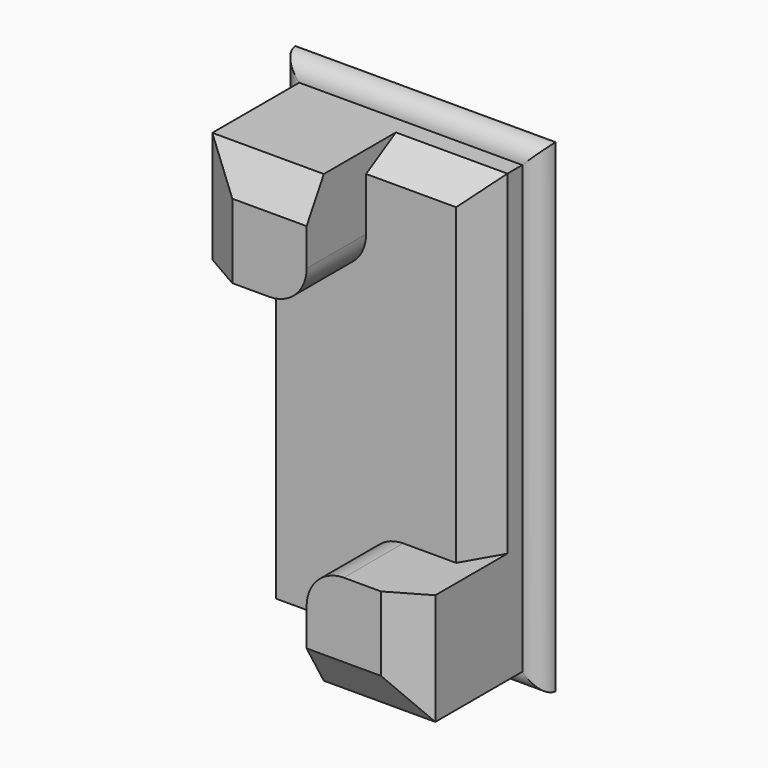
from build123d import *

# Parameters (mm, degrees)
F0_W       = 88.9
F0_H       = 165.1
F1_DEPTH   = 6.35
F2_DEPTH   = 25.4
F3_DEPTH   = 50.8
F4_SIZE2   = 7.3323484187
F4_SIZE    = 12.7
F4_2_SIZE2 = 7.3323484187
F4_2_SIZE  = 12.7
F5_R       = 6.34999
F6_SIZE2   = 7.3323484187
F6_SIZE    = 12.7
F7_SIZE2   = 7.3323484187
F7_SIZE    = 12.7


# Not quite as in the source:
# - a fillet or chamfer is up to 0.001 mm smaller than in the source, because OpenCascade refuses the exact size


with BuildPart() as f1:
    # F0 (on Front) → F1 (new body)
    with BuildSketch(Plane.XZ):
        Rectangle(F0_W, F0_H)
        Polygon((-38.1, 38.1), (-38.1, 76.2), (0, 76.2), (38.1, 76.2), (38.1, -38.1), (38.1, -76.2), (0, -76.2), (-38.1, -76.2), align=None, mode=Mode.SUBTRACT)
    extrude(amount=F1_DEPTH)

    # F0 (on Front) → F2 (join)
    with BuildSketch(Plane.XZ):
        with BuildLine():
            Line((38.1, 76.2), (0, 76.2))
            Line((0, 76.2), (0, 50.8))
            ThreePointArc((0, 50.8), (-3.7197438789, 41.8197438789), (-12.7, 38.1))
            Line((-12.7, 38.1), (-38.1, 38.1))
            Line((-38.1, 38.1), (-38.1, -76.2))
            Line((-38.1, -76.2), (0, -76.2))
            Line((0, -76.2), (0, -50.8))
            ThreePointArc((0, -50.8), (3.7197438789, -41.8197438789), (12.7, -38.1))
            Line((12.7, -38.1), (38.1, -38.1))
            Line((38.1, -38.1), (38.1, 76.2))
        make_face()
    extrude(amount=F2_DEPTH)

    # F0 (on Front) → F3 (join)
    with BuildSketch(Plane.XZ):
        with BuildLine():
            Line((0, 76.2), (-38.1, 76.2))
            Line((-38.1, 76.2), (-38.1, 38.1))
            Line((-38.1, 38.1), (-12.7, 38.1))
            ThreePointArc((-12.7, 38.1), (-3.7197438789, 41.8197438789), (0, 50.8))
            Line((0, 50.8), (0, 76.2))
        make_face()
        with BuildLine():
            Line((38.1, -76.2), (38.1, -38.1))
            Line((38.1, -38.1), (12.7, -38.1))
            ThreePointArc((12.7, -38.1), (3.7197438789, -41.8197438789), (0, -50.8))
            Line((0, -50.8), (0, -76.2))
            Line((0, -76.2), (38.1, -76.2))
        make_face()
    extrude(amount=F3_DEPTH)

    # F4
    f4_edges = [f1.edges().sort_by_distance(p)[0] for p in [
        (-38.1, -50.8, 57.15),
        (-19.05, -50.8, 76.2),
    ]]
    f4_side = f1.faces().sort_by_distance((-19.446042, -50.8, 57.546042))[0]
    chamfer(f4_edges, length=F4_SIZE, length2=F4_SIZE2, reference=f4_side)

    # F4#2
    f4_2_edges = [f1.edges().sort_by_distance(p)[0] for p in [
        (19.05, -50.8, -76.2),
    ]]
    f4_2_side = f1.faces().sort_by_distance((19.446042, -50.8, -57.546042))[0]
    chamfer(f4_2_edges, length=F4_2_SIZE, length2=F4_2_SIZE2, reference=f4_2_side)

    # F5 (radius 6.35 in the source; OpenCascade refuses exactly that, so slightly less here)
    f5_edges = [f1.edges().sort_by_distance(p)[0] for p in [
        (44.45, -6.35, 0),
        (0, -6.35, 82.55),
        (-44.45, -6.35, 0),
        (0, -6.35, -82.55),
    ]]
    fillet(f5_edges, radius=F5_R)

    # F6
    f6_edges = [f1.edges().sort_by_distance(p)[0] for p in [
        (38.1, -25.4, 19.05),
        (19.05, -25.4, 76.2),
        (-38.1, -25.4, -19.05),
        (-19.05, -25.4, -76.2),
    ]]
    chamfer(f6_edges, length=F6_SIZE, length2=F6_SIZE2)

    # F7
    f7_edges = [f1.edges().sort_by_distance(p)[0] for p in [
        (38.1, -50.8, -50.8),
    ]]
    f7_side = f1.faces().sort_by_distance((19.651409, -50.8, -51.165864))[0]
    chamfer(f7_edges, length=F7_SIZE, length2=F7_SIZE2, reference=f7_side)


solid = f1.part
